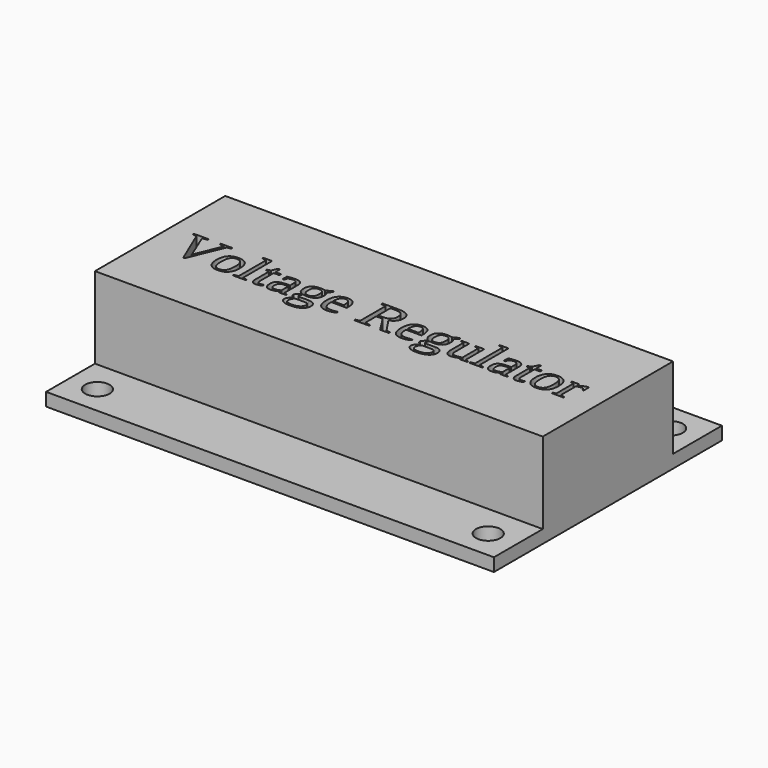
from build123d import *

# Parameters (mm, degrees)
F0_W         = 55
F0_H         = 35
F0_R         = 1.5
F1_DEPTH     = 1.6
F2_W         = 55
F2_H         = 20
F3_DEPTH     = 10
F4_TEXT_SIZE = 6.7450782008
F5_DEPTH     = 3


# Not quite as in the source:
# - Text() gives the source's letters only with a copy of the font that has no kerning and outlines rounded to 1/6400 em; it was checked with that copy


with BuildPart() as f1:
    # F0 (on Top) → F1 (new body)
    with BuildSketch(Plane.XY):
        Rectangle(F0_W, F0_H)
        with Locations((-24, -14)):
            Circle(F0_R, mode=Mode.SUBTRACT)
        with Locations((24, -14)):
            Circle(F0_R, mode=Mode.SUBTRACT)
        with Locations((-24, 14)):
            Circle(F0_R, mode=Mode.SUBTRACT)
        with Locations((24, 14)):
            Circle(F0_R, mode=Mode.SUBTRACT)
    extrude(amount=F1_DEPTH)

    # F2 (on face) → F3 (join)
    with BuildSketch(Plane.XY.offset(1.6)):
        Rectangle(F2_W, F2_H)
    extrude(amount=F3_DEPTH)

    # F4 (on face) → F5 (cut)
    with BuildSketch(Plane.XY.offset(11.6)):
        with Locations((-25, -2.4282281523)):
            Text('Voltage Regulator', F4_TEXT_SIZE, font='Tinos', text_align=(TextAlign.LEFT, TextAlign.BOTTOM))
    extrude(amount=-F5_DEPTH, mode=Mode.SUBTRACT)


solid = f1.part
